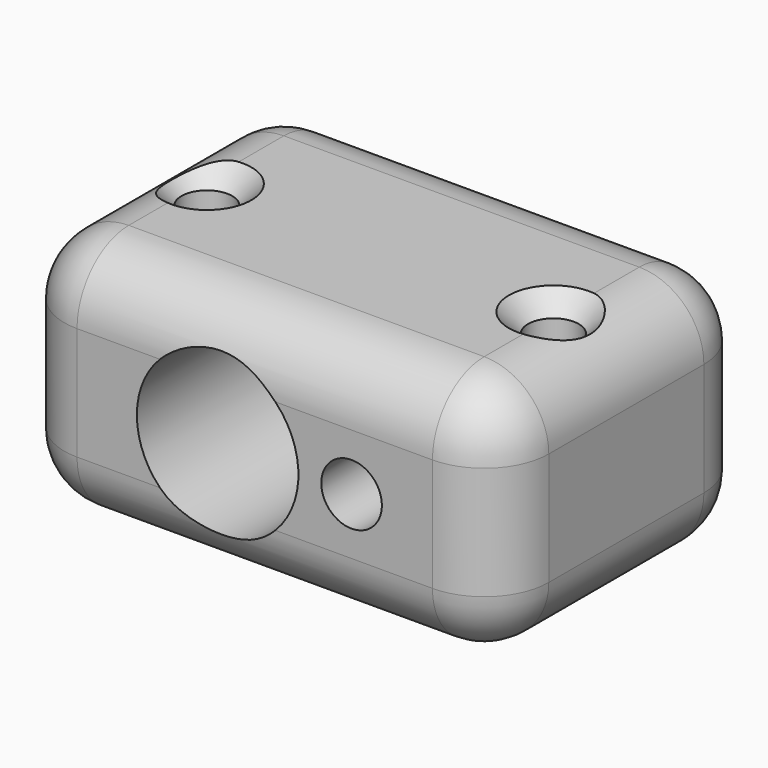
from build123d import *

# Parameters (mm, degrees)
F0_W           = 38.1
F0_H           = 19.05
F1_DEPTH       = 25.4
F2_D           = 12.7
F3_D           = 4.7625
F5_D           = 4
F5_CSINK_D     = 7
F5_CSINK_ANGLE = 90
F6_T1_DEPTH    = 27.94
F6_T3_DEPTH    = 15.24
F6_T5_DEPTH    = 8.89
F6_S9_W        = 5.08
F6_S9_H        = 5.08
F6_T10_DEPTH   = 5.08
F6_S15_W       = 5.08
F6_S15_H       = 5.08
F6_T16_DEPTH   = 5.08
F6_S21_W       = 5.08
F6_S21_H       = 5.08
F6_T22_DEPTH   = 5.08
F6_S27_W       = 5.08
F6_S27_H       = 5.08
F6_T28_DEPTH   = 5.08
F6_S33_W       = 5.08
F6_S33_H       = 5.08
F6_T34_DEPTH   = 5.08
F6_S39_W       = 5.08
F6_S39_H       = 5.08
F6_T40_DEPTH   = 5.08
F6_S45_W       = 5.08
F6_S45_H       = 5.08
F6_T46_DEPTH   = 5.08
F6_S51_W       = 5.08
F6_S51_H       = 5.08
F6_T52_DEPTH   = 5.08


# Not quite as in the source:
# - a fillet or chamfer that OpenCascade refuses, or shapes differently, is made with other operations: its cross-section is extruded or revolved along the edge and cut away or added


with BuildPart() as f1:
    # F0 (on Front) → F1 (new body)
    with BuildSketch(Plane.XZ):
        Rectangle(F0_W, F0_H)
    extrude(amount=F1_DEPTH)

    # F2 (through all)
    with Locations(Plane(origin=(0, 0, 0), x_dir=(1, 0, 0), z_dir=(0, 1, 0))):
        with Locations((-2.9169023037, 0)):
            Hole(F2_D / 2)

    # F3 (through all)
    with Locations(Plane(origin=(0, 0, 0), x_dir=(1, 0, 0), z_dir=(0, 1, 0))):
        with Locations((7.6106409542, 0)):
            Hole(F3_D / 2)

    # F5 (through all)
    with Locations(Plane.XY.offset(9.525)):
        with Locations((-13.6843686923, -12.9993055016), (13.5552566499, -12.9993055016)):
            CounterSinkHole(F5_D / 2, F5_CSINK_D / 2, counter_sink_angle=F5_CSINK_ANGLE)

    # F6: fillet of radius 5.08 on 12 edges, made by hand

    # F6_s2 → F6_t1 (cut)
    with BuildSketch(Plane.YZ.offset(-13.97)):
        with BuildLine():
            ThreePointArc((-5.08, 9.525), (-1.4878975516, 8.0371024484), (0, 4.445))
            Line((0, 4.445), (0, 9.525))
            Line((0, 9.525), (-5.08, 9.525))
        make_face()
        with BuildLine():
            ThreePointArc((-20.32, 9.525), (-23.9121024484, 8.0371024484), (-25.4, 4.445))
            Line((-25.4, 4.445), (-25.4, 9.525))
            Line((-25.4, 9.525), (-20.32, 9.525))
        make_face()
        with BuildLine():
            ThreePointArc((-20.32, -9.525), (-23.9121024484, -8.0371024484), (-25.4, -4.445))
            Line((-25.4, -4.445), (-25.4, -9.525))
            Line((-25.4, -9.525), (-20.32, -9.525))
        make_face()
        with BuildLine():
            ThreePointArc((-5.08, -9.525), (-1.4878975516, -8.0371024484), (0, -4.445))
            Line((0, -4.445), (0, -9.525))
            Line((0, -9.525), (-5.08, -9.525))
        make_face()
    extrude(amount=F6_T1_DEPTH, mode=Mode.SUBTRACT)

    # F6_s4 → F6_t3 (cut)
    with BuildSketch(Plane.XZ.offset(5.08)):
        with BuildLine():
            ThreePointArc((13.97, -9.525), (17.5621024484, -8.0371024484), (19.05, -4.445))
            Line((19.05, -4.445), (19.05, -9.525))
            Line((19.05, -9.525), (13.97, -9.525))
        make_face()
        with BuildLine():
            ThreePointArc((13.97, 9.525), (17.5621024484, 8.0371024484), (19.05, 4.445))
            Line((19.05, 4.445), (19.05, 9.525))
            Line((19.05, 9.525), (13.97, 9.525))
        make_face()
        with BuildLine():
            ThreePointArc((-19.05, 4.445), (-17.5621024484, 8.0371024484), (-13.97, 9.525))
            Line((-13.97, 9.525), (-19.05, 9.525))
            Line((-19.05, 9.525), (-19.05, 4.445))
        make_face()
        with BuildLine():
            ThreePointArc((-19.05, -4.445), (-17.5621024484, -8.0371024484), (-13.97, -9.525))
            Line((-13.97, -9.525), (-19.05, -9.525))
            Line((-19.05, -9.525), (-19.05, -4.445))
        make_face()
    extrude(amount=F6_T3_DEPTH, mode=Mode.SUBTRACT)

    # F6_s6 → F6_t5 (cut)
    with BuildSketch(Plane.XY.offset(-4.445)):
        with BuildLine():
            ThreePointArc((13.97, 0), (17.5621024484, -1.4878975516), (19.05, -5.08))
            Line((19.05, -5.08), (19.05, 0))
            Line((19.05, 0), (13.97, 0))
        make_face()
        with BuildLine():
            ThreePointArc((13.97, -25.4), (17.5621024484, -23.9121024484), (19.05, -20.32))
            Line((19.05, -20.32), (19.05, -25.4))
            Line((19.05, -25.4), (13.97, -25.4))
        make_face()
        with BuildLine():
            ThreePointArc((-19.05, -5.08), (-17.5621024484, -1.4878975516), (-13.97, 0))
            Line((-13.97, 0), (-19.05, 0))
            Line((-19.05, 0), (-19.05, -5.08))
        make_face()
        with BuildLine():
            ThreePointArc((-19.05, -20.32), (-17.5621024484, -23.9121024484), (-13.97, -25.4))
            Line((-13.97, -25.4), (-19.05, -25.4))
            Line((-19.05, -25.4), (-19.05, -20.32))
        make_face()
    extrude(amount=F6_T5_DEPTH, mode=Mode.SUBTRACT)


with BuildPart() as f6_tool8:
    # F6_s9 → F6_t10 (new body)
    with BuildSketch(Plane.XY.offset(4.445)):
        with Locations((16.51, -2.54)):
            Rectangle(F6_S9_W, F6_S9_H)
    extrude(amount=F6_T10_DEPTH)

    # F6_s11 → F6_t12 (revolve, cut)
    with BuildSketch(Plane(origin=(13.97, -5.08, 4.445), x_dir=(-0.7071067812, -0.7071067812, 0), z_dir=(-0.7071067812, 0.7071067812, 0))):
        with BuildLine():
            ThreePointArc((0, -5.08), (5.08, 0), (0, 5.08))
            Line((0, 5.08), (0, -5.08))
        make_face()
    revolve(axis=Axis((13.97, -5.08, 4.445), (0, 0, 1)), mode=Mode.SUBTRACT)


with BuildPart() as f1_1:
    add(f1.part)

    # F6_t7: cut F6_tool8
    add(f6_tool8.part, mode=Mode.SUBTRACT)


with BuildPart() as f6_tool14:
    # F6_s15 → F6_t16 (new body)
    with BuildSketch(Plane.YZ.offset(-13.97)):
        with Locations((-2.54, 6.985)):
            Rectangle(F6_S15_W, F6_S15_H)
    extrude(amount=-F6_T16_DEPTH)

    # F6_s17 → F6_t18 (revolve, cut)
    with BuildSketch(Plane(origin=(-13.97, -5.08, 4.445), x_dir=(0, -0.7071067812, -0.7071067812), z_dir=(0, 0.7071067812, -0.7071067812))):
        with BuildLine():
            ThreePointArc((0, -5.08), (5.08, 0), (0, 5.08))
            Line((0, 5.08), (0, -5.08))
        make_face()
    revolve(axis=Axis((-13.97, -5.08, 4.445), (-1, 0, 0)), mode=Mode.SUBTRACT)


with BuildPart() as f1_2:
    add(f1_1.part)

    # F6_t13: cut F6_tool14
    add(f6_tool14.part, mode=Mode.SUBTRACT)


with BuildPart() as f6_tool20:
    # F6_s21 → F6_t22 (new body)
    with BuildSketch(Plane.XY.offset(4.445)):
        with Locations((16.51, -22.86)):
            Rectangle(F6_S21_W, F6_S21_H)
    extrude(amount=F6_T22_DEPTH)

    # F6_s23 → F6_t24 (revolve, cut)
    with BuildSketch(Plane(origin=(13.97, -20.32, 4.445), x_dir=(-0.7071067812, 0.7071067812, 0), z_dir=(0.7071067812, 0.7071067812, 0))):
        with BuildLine():
            ThreePointArc((0, -5.08), (5.08, 0), (0, 5.08))
            Line((0, 5.08), (0, -5.08))
        make_face()
    revolve(axis=Axis((13.97, -20.32, 4.445), (0, 0, 1)), mode=Mode.SUBTRACT)


with BuildPart() as f1_3:
    add(f1_2.part)

    # F6_t19: cut F6_tool20
    add(f6_tool20.part, mode=Mode.SUBTRACT)


with BuildPart() as f6_tool26:
    # F6_s27 → F6_t28 (new body)
    with BuildSketch(Plane.YZ.offset(-13.97)):
        with Locations((-22.86, 6.985)):
            Rectangle(F6_S27_W, F6_S27_H)
    extrude(amount=-F6_T28_DEPTH)

    # F6_s29 → F6_t30 (revolve, cut)
    with BuildSketch(Plane(origin=(-13.97, -20.32, 4.445), x_dir=(0, 0.7071067812, -0.7071067812), z_dir=(0, 0.7071067812, 0.7071067812))):
        with BuildLine():
            ThreePointArc((0, -5.08), (5.08, 0), (0, 5.08))
            Line((0, 5.08), (0, -5.08))
        make_face()
    revolve(axis=Axis((-13.97, -20.32, 4.445), (-1, 0, 0)), mode=Mode.SUBTRACT)


with BuildPart() as f1_4:
    add(f1_3.part)

    # F6_t25: cut F6_tool26
    add(f6_tool26.part, mode=Mode.SUBTRACT)


with BuildPart() as f6_tool32:
    # F6_s33 → F6_t34 (new body)
    with BuildSketch(Plane.YZ.offset(-13.97)):
        with Locations((-22.86, -6.985)):
            Rectangle(F6_S33_W, F6_S33_H)
    extrude(amount=-F6_T34_DEPTH)

    # F6_s35 → F6_t36 (revolve, cut)
    with BuildSketch(Plane(origin=(-13.97, -20.32, -4.445), x_dir=(0, 0.7071067812, 0.7071067812), z_dir=(0, -0.7071067812, 0.7071067812))):
        with BuildLine():
            ThreePointArc((0, -5.08), (5.08, 0), (0, 5.08))
            Line((0, 5.08), (0, -5.08))
        make_face()
    revolve(axis=Axis((-13.97, -20.32, -4.445), (-1, 0, 0)), mode=Mode.SUBTRACT)


with BuildPart() as f1_5:
    add(f1_4.part)

    # F6_t31: cut F6_tool32
    add(f6_tool32.part, mode=Mode.SUBTRACT)


with BuildPart() as f6_tool38:
    # F6_s39 → F6_t40 (new body)
    with BuildSketch(Plane.XY.offset(-4.445)):
        with Locations((16.51, -22.86)):
            Rectangle(F6_S39_W, F6_S39_H)
    extrude(amount=-F6_T40_DEPTH)

    # F6_s41 → F6_t42 (revolve, cut)
    with BuildSketch(Plane(origin=(13.97, -20.32, -4.445), x_dir=(-0.7071067812, 0.7071067812, 0), z_dir=(-0.7071067812, -0.7071067812, 0))):
        with BuildLine():
            ThreePointArc((0, -5.08), (5.08, 0), (0, 5.08))
            Line((0, 5.08), (0, -5.08))
        make_face()
    revolve(axis=Axis((13.97, -20.32, -4.445), (0, 0, -1)), mode=Mode.SUBTRACT)


with BuildPart() as f1_6:
    add(f1_5.part)

    # F6_t37: cut F6_tool38
    add(f6_tool38.part, mode=Mode.SUBTRACT)


with BuildPart() as f6_tool44:
    # F6_s45 → F6_t46 (new body)
    with BuildSketch(Plane.YZ.offset(-13.97)):
        with Locations((-2.54, -6.985)):
            Rectangle(F6_S45_W, F6_S45_H)
    extrude(amount=-F6_T46_DEPTH)

    # F6_s47 → F6_t48 (revolve, cut)
    with BuildSketch(Plane(origin=(-13.97, -5.08, -4.445), x_dir=(0, -0.7071067812, 0.7071067812), z_dir=(0, -0.7071067812, -0.7071067812))):
        with BuildLine():
            ThreePointArc((0, -5.08), (5.08, 0), (0, 5.08))
            Line((0, 5.08), (0, -5.08))
        make_face()
    revolve(axis=Axis((-13.97, -5.08, -4.445), (-1, 0, 0)), mode=Mode.SUBTRACT)


with BuildPart() as f1_7:
    add(f1_6.part)

    # F6_t43: cut F6_tool44
    add(f6_tool44.part, mode=Mode.SUBTRACT)


with BuildPart() as f6_tool50:
    # F6_s51 → F6_t52 (new body)
    with BuildSketch(Plane.XY.offset(-4.445)):
        with Locations((16.51, -2.54)):
            Rectangle(F6_S51_W, F6_S51_H)
    extrude(amount=-F6_T52_DEPTH)

    # F6_s53 → F6_t54 (revolve, cut)
    with BuildSketch(Plane(origin=(13.97, -5.08, -4.445), x_dir=(-0.7071067812, -0.7071067812, 0), z_dir=(0.7071067812, -0.7071067812, 0))):
        with BuildLine():
            ThreePointArc((0, -5.08), (5.08, 0), (0, 5.08))
            Line((0, 5.08), (0, -5.08))
        make_face()
    revolve(axis=Axis((13.97, -5.08, -4.445), (0, 0, -1)), mode=Mode.SUBTRACT)


with BuildPart() as f1_8:
    add(f1_7.part)

    # F6_t49: cut F6_tool50
    add(f6_tool50.part, mode=Mode.SUBTRACT)


solid = f1_8.part
